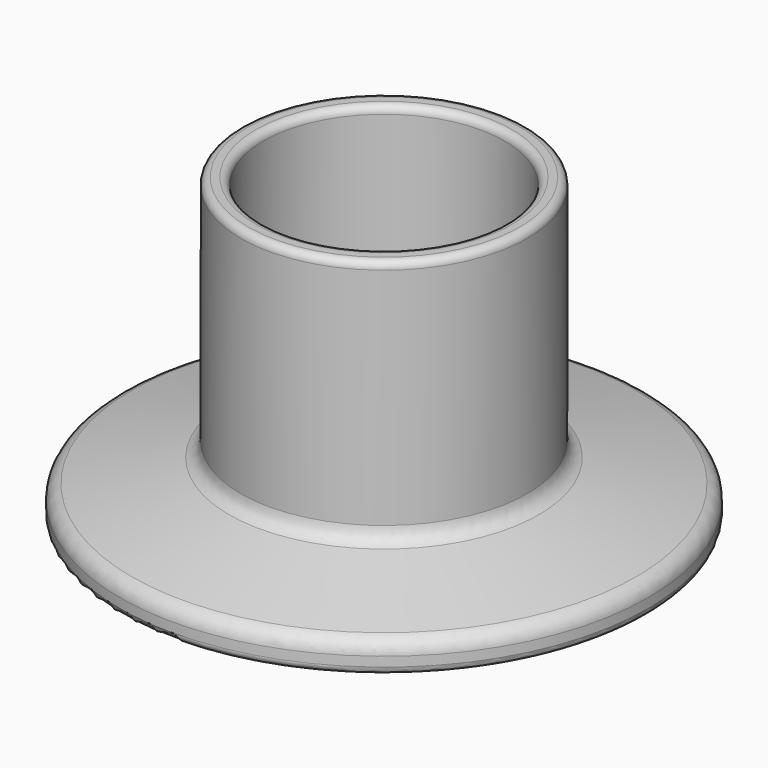
from build123d import *

# Parameters (mm, degrees)
F2_SIZE = 1.99999
F3_R    = 2
F4_R    = 1
F5_SIZE = 1.99999


# Not quite as in the source:
# - a fillet or chamfer is up to 0.001 mm smaller than in the source, because OpenCascade refuses the exact size


with BuildPart() as f1:
    # F0 (on Front) → F1 (revolve)
    with BuildSketch(Plane.XZ):
        Polygon((-35, 0), (-32, 0), (-32, 1.4718503955), (-16, 5.2344552971), (-16, 12), (-14, 12), (-14, 15), (-16, 15), (-16, 40), (-19, 40), (-19, 7.6108030044), (-35, 3.8481981028), align=None)
    revolve(axis=Axis((0, 0, 9.703790769), (0, 0, -1)))

    # F2 (size 2 in the source; OpenCascade refuses exactly that, so slightly less here)
    f2_edges = [f1.edges().sort_by_distance(p)[0] for p in [
        (16, 0, 15),
    ]]
    chamfer(f2_edges, length=F2_SIZE)

    # F3
    f3_edges = [f1.edges().sort_by_distance(p)[0] for p in [
        (35, 0, 3.848198),
        (19, 0, 7.610803),
    ]]
    fillet(f3_edges, radius=F3_R)

    # F4
    f4_edges = [f1.edges().sort_by_distance(p)[0] for p in [
        (32, 0, 1.47185),
        (16, 0, 5.234455),
        (35, 0, 0),
        (19, 0, 40),
        (16, 0, 40),
    ]]
    fillet(f4_edges, radius=F4_R)

    # F5 (size 2 in the source; OpenCascade refuses exactly that, so slightly less here)
    f5_edges = [f1.edges().sort_by_distance(p)[0] for p in [
        (16, 0, 12),
    ]]
    chamfer(f5_edges, length=F5_SIZE)


solid = f1.part
